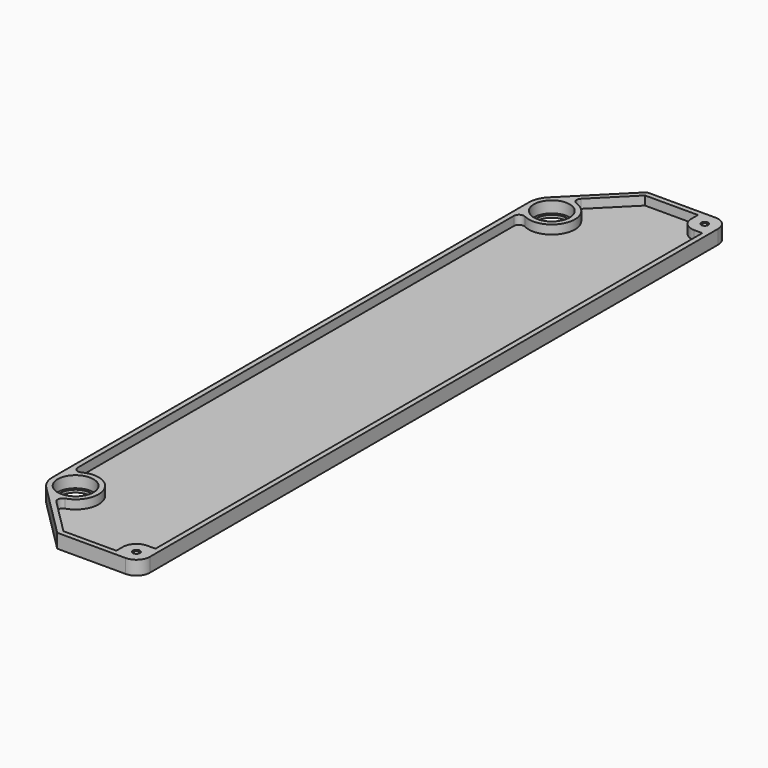
from build123d import *

# Parameters (mm, degrees)
F0_R      = 9.525
F1_DEPTH  = 8.6995
F2_R      = 11.1125
F3_DEPTH  = 7.112
F4_T      = -3.175
F5_R      = 3.175
F6_W      = 16.66875
F6_H      = 16.66875
F7_DEPTH  = 5.5245
F8_R      = 8.334375
F9_R      = 6.746875
F10_DEPTH = 7.9375
F11_R     = 2.15265
F12_DEPTH = 8.6995


with BuildPart() as f1:
    # F0 (on Top) → F1 (new body)
    with BuildSketch(Plane.XY):
        with BuildLine():
            Line((-14.2875, 369.1638474552), (-14.2875, 0))
            ThreePointArc((-14.2875, 0), (-13.1999288208, -5.4675895399), (-10.1027881362, -10.1027881362))
            Line((-10.1027881362, -10.1027881362), (23.8125, -44.0180762724))
            Line((23.8125, -44.0180762724), (74.6125, -44.0180762724))
            Line((74.6125, -44.0180762724), (74.6125, 413.1819237276))
            Line((74.6125, 413.1819237276), (23.8125, 413.1819237276))
            Line((23.8125, 413.1819237276), (-10.1027881362, 379.2666355914))
            ThreePointArc((-10.1027881362, 379.2666355914), (-13.1999288208, 374.6314369951), (-14.2875, 369.1638474552))
        make_face()
        Circle(F0_R, mode=Mode.SUBTRACT)
        with Locations((0, 369.1638474552)):
            Circle(F0_R, mode=Mode.SUBTRACT)
    extrude(amount=F1_DEPTH)

    # F2 (on face) → F3 (cut)
    with BuildSketch(Plane.XY.offset(8.6995)):
        with Locations((0, 369.1638474552)):
            Circle(F2_R)
        Circle(F2_R)
    extrude(amount=-F3_DEPTH, mode=Mode.SUBTRACT)

    # F4
    f4_openings = [f1.faces().sort_by_distance(p)[0] for p in [
        (31.981731, 184.581924, 8.6995),
    ]]
    offset(amount=F4_T, openings=f4_openings)

    # F5
    f5_edges = [f1.edges().sort_by_distance(p)[0] for p in [
        (-1.507724, 383.371572, 5.93725),
        (-11.1125, 360.183591, 5.93725),
        (-11.1125, 8.980256, 5.93725),
        (-1.507724, -14.207724, 5.93725),
    ]]
    fillet(f5_edges, radius=F5_R)

    # F6 (on face) → F7 (join, through all)
    with BuildSketch(Plane.XY.offset(3.175)):
        with Locations((66.278125, 404.8475487276)):
            Rectangle(F6_W, F6_H)
        with Locations((66.278125, -35.6837012724)):
            Rectangle(F6_W, F6_H)
    extrude(amount=F7_DEPTH)

    # F8
    f8_edges = [f1.edges().sort_by_distance(p)[0] for p in [
        (74.6125, 413.181924, 4.34975),
        (74.6125, -44.018076, 4.34975),
        (57.94375, -27.349326, 5.93725),
        (57.94375, 396.513174, 5.93725),
    ]]
    fillet(f8_edges, radius=F8_R)

    # F9 (on face) → F10 (cut)
    with BuildSketch(Plane(origin=(0, 0, 0), x_dir=(1, 0, 0), z_dir=(0, 0, -1))):
        with Locations((66.278125, 35.6837012724)):
            Circle(F9_R)
        with Locations((66.278125, -404.8475487276)):
            Circle(F9_R)
    extrude(amount=-F10_DEPTH, mode=Mode.SUBTRACT)

    # F11 (on face) → F12 (cut, through all)
    with BuildSketch(Plane(origin=(0, 0, 0), x_dir=(1, 0, 0), z_dir=(0, 0, -1))):
        with Locations((66.278125, 35.6837012724)):
            Circle(F11_R)
        with Locations((66.278125, -404.8475487276)):
            Circle(F11_R)
    extrude(amount=-F12_DEPTH, mode=Mode.SUBTRACT)


solid = f1.part
